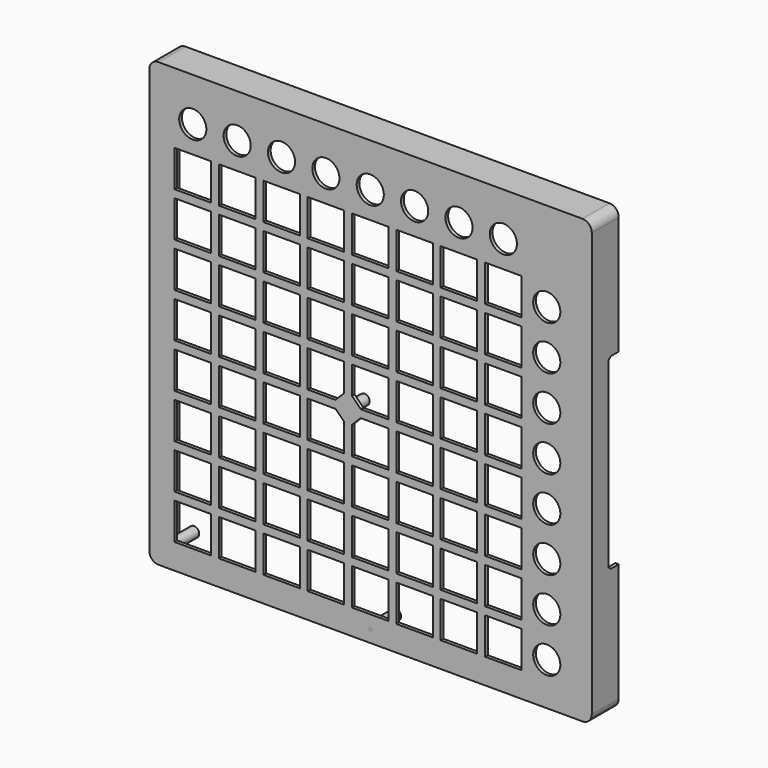
from build123d import *

# Parameters (mm, degrees)
F1_DEPTH  = 18
F0_R      = 2.75
F0_W      = 19.5
F0_H      = 19.5
F0_R_2    = 7.25
F2_DEPTH  = 1.8
F0_R_3    = 0.9
F3_DEPTH  = 17
F4_DEPTH  = 1.8
F0_R_4    = 0.875
F5_DEPTH  = 1.8
F6_DEPTH  = 17
F7_DEPTH  = 1.8
F8_DEPTH  = 17
F9_DEPTH  = 1.8
F10_DEPTH = 17
F12_DEPTH = 325
F13_DEPTH = 17
F14_DEPTH = 1.8
F15_DEPTH = 17
F16_DEPTH = 1.8
F17_W     = 1.5
F17_H     = 11.8
F18_W     = 1.5
F18_H     = 11.8
F19_DEPTH = 0.5
F20_R     = 0.49999


# Not quite as in the source:
# - a fillet or chamfer is up to 0.001 mm smaller than in the source, because OpenCascade refuses the exact size


with BuildPart() as f1:
    # F0 (on Front) → F1 (new body)
    with BuildSketch(Plane.XZ):
        with BuildLine():
            Line((-113.2, -118.2), (113.2, -118.2))
            ThreePointArc((113.2, -118.2), (116.7355339059, -116.7355339059), (118.2, -113.2))
            Line((118.2, -113.2), (118.2, 113.2))
            ThreePointArc((118.2, 113.2), (116.7355339059, 116.7355339059), (113.2, 118.2))
            Line((113.2, 118.2), (-113.2, 118.2))
            ThreePointArc((-113.2, 118.2), (-116.7355339059, 116.7355339059), (-118.2, 113.2))
            Line((-118.2, 113.2), (-118.2, -113.2))
            ThreePointArc((-118.2, -113.2), (-116.7355339059, -116.7355339059), (-113.2, -118.2))
        make_face()
        with BuildLine():
            ThreePointArc((116.4, -111.4), (114.9355339059, -114.9355339059), (111.4, -116.4))
            Line((111.4, -116.4), (-111.4, -116.4))
            ThreePointArc((-111.4, -116.4), (-114.9355339059, -114.9355339059), (-116.4, -111.4))
            Line((-116.4, -111.4), (-116.4, 111.4))
            ThreePointArc((-116.4, 111.4), (-114.9355339059, 114.9355339059), (-111.4, 116.4))
            Line((-111.4, 116.4), (111.4, 116.4))
            ThreePointArc((111.4, 116.4), (114.9355339059, 114.9355339059), (116.4, 111.4))
            Line((116.4, 111.4), (116.4, -111.4))
        make_face(mode=Mode.SUBTRACT)
    extrude(amount=-F1_DEPTH)

    # F0 (on Front) → F2 (join)
    with BuildSketch(Plane.XZ):
        with BuildLine():
            Line((-111.4, -116.4), (111.4, -116.4))
            ThreePointArc((111.4, -116.4), (114.9355339059, -114.9355339059), (116.4, -111.4))
            Line((116.4, -111.4), (116.4, 111.4))
            ThreePointArc((116.4, 111.4), (114.9355339059, 114.9355339059), (111.4, 116.4))
            Line((111.4, 116.4), (-111.4, 116.4))
            ThreePointArc((-111.4, 116.4), (-114.9355339059, 114.9355339059), (-116.4, 111.4))
            Line((-116.4, 111.4), (-116.4, -111.4))
            ThreePointArc((-116.4, -111.4), (-114.9355339059, -114.9355339059), (-111.4, -116.4))
        make_face()
        with Locations((-107.85, -107.85)):
            Circle(F0_R, mode=Mode.SUBTRACT)
        with Locations((-94.95, -94.95)):
            Rectangle(F0_W, F0_H, mode=Mode.SUBTRACT)
        with Locations((-71.25, -94.95)):
            Rectangle(F0_W, F0_H, mode=Mode.SUBTRACT)
        with Locations((-94.95, -71.25)):
            Rectangle(F0_W, F0_H, mode=Mode.SUBTRACT)
        with Locations((-71.25, -71.25)):
            Rectangle(F0_W, F0_H, mode=Mode.SUBTRACT)
        with Locations((-47.55, -94.95)):
            Rectangle(F0_W, F0_H, mode=Mode.SUBTRACT)
        with Locations((-23.85, -94.95)):
            Rectangle(F0_W, F0_H, mode=Mode.SUBTRACT)
        with Locations((-0.1497857198, -94.95)):
            Rectangle(F0_W, F0_H, mode=Mode.SUBTRACT)
        with Locations((-47.55, -71.25)):
            Rectangle(F0_W, F0_H, mode=Mode.SUBTRACT)
        with Locations((-23.85, -71.25)):
            Rectangle(F0_W, F0_H, mode=Mode.SUBTRACT)
        with Locations((-0.1497857198, -71.25)):
            Rectangle(F0_W, F0_H, mode=Mode.SUBTRACT)
        with Locations((-94.95, -47.55)):
            Rectangle(F0_W, F0_H, mode=Mode.SUBTRACT)
        with Locations((-71.25, -47.55)):
            Rectangle(F0_W, F0_H, mode=Mode.SUBTRACT)
        with Locations((-94.95, -23.85)):
            Rectangle(F0_W, F0_H, mode=Mode.SUBTRACT)
        with Locations((-94.95, -0.15)):
            Rectangle(F0_W, F0_H, mode=Mode.SUBTRACT)
        with Locations((-71.25, -23.85)):
            Rectangle(F0_W, F0_H, mode=Mode.SUBTRACT)
        with Locations((-71.25, -0.15)):
            Rectangle(F0_W, F0_H, mode=Mode.SUBTRACT)
        with Locations((-47.55, -47.55)):
            Rectangle(F0_W, F0_H, mode=Mode.SUBTRACT)
        with Locations((-23.85, -47.55)):
            Rectangle(F0_W, F0_H, mode=Mode.SUBTRACT)
        with Locations((-0.1497857198, -47.55)):
            Rectangle(F0_W, F0_H, mode=Mode.SUBTRACT)
        with Locations((-47.55, -23.85)):
            Rectangle(F0_W, F0_H, mode=Mode.SUBTRACT)
        with Locations((-47.55, -0.15)):
            Rectangle(F0_W, F0_H, mode=Mode.SUBTRACT)
        Polygon((9.6002142802, 9.6), (9.6002142802, -9.9), (-5.1834957055, -9.9), (-3.1223304703, -11.9611652352), (-5.2611652352, -14.1), (9.6002142802, -14.1), (9.6002142802, -33.6), (-9.8997857198, -33.6), (-9.8997857198, -18.7386204846), (-11.9611652352, -20.8), (-14.1, -18.6611652352), (-14.1, -33.6), (-33.6, -33.6), (-33.6, -14.1), (-18.6611652352, -14.1), (-20.8, -11.9611652352), (-18.7388347648, -9.9), (-33.6, -9.9), (-33.6, 9.6), (-14.1, 9.6), (-14.1, -5.2611652352), (-11.9611652352, -3.1223304703), (-9.8997857198, -5.1837099858), (-9.8997857198, 9.6), align=None, mode=Mode.SUBTRACT)
        with Locations((0, -111.65)):
            Circle(F0_R, mode=Mode.SUBTRACT)
        with Locations((23.55, -94.95)):
            Rectangle(F0_W, F0_H, mode=Mode.SUBTRACT)
        with Locations((47.25, -94.95)):
            Rectangle(F0_W, F0_H, mode=Mode.SUBTRACT)
        with Locations((23.55, -71.25)):
            Rectangle(F0_W, F0_H, mode=Mode.SUBTRACT)
        with Locations((47.25, -71.25)):
            Rectangle(F0_W, F0_H, mode=Mode.SUBTRACT)
        with Locations((70.95, -94.95)):
            Rectangle(F0_W, F0_H, mode=Mode.SUBTRACT)
        with Locations((107.85, -107.85)):
            Circle(F0_R, mode=Mode.SUBTRACT)
        with Locations((94.15, -95.45)):
            Circle(F0_R_2, mode=Mode.SUBTRACT)
        with Locations((70.95, -71.25)):
            Rectangle(F0_W, F0_H, mode=Mode.SUBTRACT)
        with Locations((94.1499999885, -71.75)):
            Circle(F0_R_2, mode=Mode.SUBTRACT)
        with Locations((23.55, -47.55)):
            Rectangle(F0_W, F0_H, mode=Mode.SUBTRACT)
        with Locations((47.25, -47.55)):
            Rectangle(F0_W, F0_H, mode=Mode.SUBTRACT)
        with Locations((23.55, -23.85)):
            Rectangle(F0_W, F0_H, mode=Mode.SUBTRACT)
        with Locations((23.55, -0.15)):
            Rectangle(F0_W, F0_H, mode=Mode.SUBTRACT)
        with Locations((47.25, -23.85)):
            Rectangle(F0_W, F0_H, mode=Mode.SUBTRACT)
        with Locations((47.25, -0.15)):
            Rectangle(F0_W, F0_H, mode=Mode.SUBTRACT)
        with Locations((70.95, -47.55)):
            Rectangle(F0_W, F0_H, mode=Mode.SUBTRACT)
        with Locations((94.1499999893, -48.05)):
            Circle(F0_R_2, mode=Mode.SUBTRACT)
        with Locations((70.95, -23.85)):
            Rectangle(F0_W, F0_H, mode=Mode.SUBTRACT)
        with Locations((70.95, -0.15)):
            Rectangle(F0_W, F0_H, mode=Mode.SUBTRACT)
        with Locations((94.15, -24.35)):
            Circle(F0_R_2, mode=Mode.SUBTRACT)
        with Locations((94.15, -0.65)):
            Circle(F0_R_2, mode=Mode.SUBTRACT)
        with Locations((-94.95, 23.55)):
            Rectangle(F0_W, F0_H, mode=Mode.SUBTRACT)
        with Locations((-71.25, 23.55)):
            Rectangle(F0_W, F0_H, mode=Mode.SUBTRACT)
        with Locations((-94.95, 47.25)):
            Rectangle(F0_W, F0_H, mode=Mode.SUBTRACT)
        with Locations((-71.25, 47.25)):
            Rectangle(F0_W, F0_H, mode=Mode.SUBTRACT)
        with Locations((-47.55, 23.55)):
            Rectangle(F0_W, F0_H, mode=Mode.SUBTRACT)
        with Locations((-23.85, 23.55)):
            Rectangle(F0_W, F0_H, mode=Mode.SUBTRACT)
        with Locations((-0.1497857198, 23.55)):
            Rectangle(F0_W, F0_H, mode=Mode.SUBTRACT)
        with Locations((-47.55, 47.25)):
            Rectangle(F0_W, F0_H, mode=Mode.SUBTRACT)
        with Locations((-23.85, 47.25)):
            Rectangle(F0_W, F0_H, mode=Mode.SUBTRACT)
        with Locations((-0.15, 47.25)):
            Rectangle(F0_W, F0_H, mode=Mode.SUBTRACT)
        with Locations((-94.95, 70.95)):
            Rectangle(F0_W, F0_H, mode=Mode.SUBTRACT)
        with Locations((-71.25, 70.95)):
            Rectangle(F0_W, F0_H, mode=Mode.SUBTRACT)
        with Locations((-94.95, 94.95)):
            Circle(F0_R_2, mode=Mode.SUBTRACT)
        with Locations((-107.85, 107.85)):
            Circle(F0_R, mode=Mode.SUBTRACT)
        with Locations((-71.25, 94.95)):
            Circle(F0_R_2, mode=Mode.SUBTRACT)
        with Locations((-47.55, 70.95)):
            Rectangle(F0_W, F0_H, mode=Mode.SUBTRACT)
        with Locations((-23.85, 70.95)):
            Rectangle(F0_W, F0_H, mode=Mode.SUBTRACT)
        with Locations((-0.15, 70.95)):
            Rectangle(F0_W, F0_H, mode=Mode.SUBTRACT)
        with Locations((-47.55, 94.9499985917)):
            Circle(F0_R_2, mode=Mode.SUBTRACT)
        with Locations((-23.85, 94.9499985917)):
            Circle(F0_R_2, mode=Mode.SUBTRACT)
        with Locations((-0.15, 94.95)):
            Circle(F0_R_2, mode=Mode.SUBTRACT)
        with Locations((23.55, 23.55)):
            Rectangle(F0_W, F0_H, mode=Mode.SUBTRACT)
        with Locations((47.25, 23.55)):
            Rectangle(F0_W, F0_H, mode=Mode.SUBTRACT)
        with Locations((23.55, 47.25)):
            Rectangle(F0_W, F0_H, mode=Mode.SUBTRACT)
        with Locations((47.25, 47.25)):
            Rectangle(F0_W, F0_H, mode=Mode.SUBTRACT)
        with Locations((70.95, 23.55)):
            Rectangle(F0_W, F0_H, mode=Mode.SUBTRACT)
        with Locations((94.1499999896, 23.05)):
            Circle(F0_R_2, mode=Mode.SUBTRACT)
        with Locations((70.95, 47.25)):
            Rectangle(F0_W, F0_H, mode=Mode.SUBTRACT)
        with Locations((94.15, 46.75)):
            Circle(F0_R_2, mode=Mode.SUBTRACT)
        with Locations((23.55, 70.95)):
            Rectangle(F0_W, F0_H, mode=Mode.SUBTRACT)
        with Locations((47.25, 70.95)):
            Rectangle(F0_W, F0_H, mode=Mode.SUBTRACT)
        with Locations((23.55, 94.95)):
            Circle(F0_R_2, mode=Mode.SUBTRACT)
        with Locations((0, 111.65)):
            Circle(F0_R, mode=Mode.SUBTRACT)
        with Locations((47.25, 94.95)):
            Circle(F0_R_2, mode=Mode.SUBTRACT)
        with Locations((70.95, 70.95)):
            Rectangle(F0_W, F0_H, mode=Mode.SUBTRACT)
        with Locations((94.15, 70.45)):
            Circle(F0_R_2, mode=Mode.SUBTRACT)
        with Locations((70.95, 94.95)):
            Circle(F0_R_2, mode=Mode.SUBTRACT)
        with Locations((107.85, 107.85)):
            Circle(F0_R, mode=Mode.SUBTRACT)
        Polygon((-14.1, -9.9), (-14.1, -5.2611652352), (-18.7388347648, -9.9), align=None)
        Polygon((-3.1223304703, -11.9611652352), (-5.1834957055, -9.9), (-9.8997857198, -9.9), (-9.8997857198, -5.1837099858), (-11.9611652352, -3.1223304703), (-14.1, -5.2611652352), (-14.1, -9.9), (-18.7388347648, -9.9), (-20.8, -11.9611652352), (-18.6611652352, -14.1), (-14.1, -14.1), (-14.1, -18.6611652352), (-11.9611652352, -20.8), (-9.8997857198, -18.7386204846), (-9.8997857198, -14.1), (-5.2611652352, -14.1), align=None)
        with Locations((-12, -12)):
            Circle(F0_R, mode=Mode.SUBTRACT)
        Polygon((-18.6611652352, -14.1), (-14.1, -18.6611652352), (-14.1, -14.1), align=None)
        Polygon((-9.8997857198, -18.7386204846), (-5.2611652352, -14.1), (-9.8997857198, -14.1), align=None)
        Polygon((-9.8997857198, -9.9), (-5.1834957055, -9.9), (-9.8997857198, -5.1837099858), align=None)
    extrude(amount=-F2_DEPTH)

    # F0 (on Front) → F3 (join)
    with BuildSketch(Plane.XZ):
        with Locations((-12, -12)):
            Circle(F0_R)
        with Locations((-12, -12)):
            Circle(F0_R_3, mode=Mode.SUBTRACT)
    extrude(amount=-F3_DEPTH)

    # F0 (on Front) → F4 (join)
    with BuildSketch(Plane.XZ):
        with Locations((-12, -12)):
            Circle(F0_R_3)
    extrude(amount=-F4_DEPTH)

    # F0 (on Front) → F6 (join)
    with BuildSketch(Plane.XZ):
        with Locations((0, 111.65)):
            Circle(F0_R)
        with Locations((0, 111.65)):
            Circle(F0_R_4, mode=Mode.SUBTRACT)
    extrude(amount=-F6_DEPTH)

    # F0 (on Front) → F7 (join)
    with BuildSketch(Plane.XZ):
        with Locations((0, 111.65)):
            Circle(F0_R_4)
    extrude(amount=-F7_DEPTH)

    # F0 (on Front) → F8 (join)
    with BuildSketch(Plane.XZ):
        with Locations((107.85, -107.85)):
            Circle(F0_R)
        with Locations((107.85, -107.85)):
            Circle(F0_R_4, mode=Mode.SUBTRACT)
    extrude(amount=-F8_DEPTH)

    # F0 (on Front) → F9 (join)
    with BuildSketch(Plane.XZ):
        with Locations((107.85, -107.85)):
            Circle(F0_R_4)
    extrude(amount=-F9_DEPTH)

    # F0 (on Front) → F10 (join)
    with BuildSketch(Plane.XZ):
        with Locations((0, -111.65)):
            Circle(F0_R)
        with Locations((0, -111.65)):
            Circle(F0_R_4, mode=Mode.SUBTRACT)
    extrude(amount=-F10_DEPTH)

    # F11 (on face) → F12 (cut)
    with BuildSketch(Plane.YZ.offset(118.2)):
        with BuildLine():
            Line((18, -50), (18, 50))
            Line((18, 50), (13.5, 50))
            ThreePointArc((13.5, 50), (11.732233047, 49.267766953), (11, 47.5))
            Line((11, 47.5), (11, -47.5))
            ThreePointArc((11, -47.5), (11.732233047, -49.267766953), (13.5, -50))
            Line((13.5, -50), (18, -50))
        make_face()
    extrude(amount=-F12_DEPTH, mode=Mode.SUBTRACT)

    # F0 (on Front) → F13 (join)
    with BuildSketch(Plane.XZ):
        with Locations((107.85, 107.85)):
            Circle(F0_R)
        with Locations((107.85, 107.85)):
            Circle(F0_R_4, mode=Mode.SUBTRACT)
    extrude(amount=-F13_DEPTH)

    # F0 (on Front) → F14 (join)
    with BuildSketch(Plane.XZ):
        with Locations((107.85, 107.85)):
            Circle(F0_R_4)
    extrude(amount=-F14_DEPTH)

    # F0 (on Front) → F15 (join)
    with BuildSketch(Plane.XZ):
        with Locations((-107.85, -107.85)):
            Circle(F0_R)
        with Locations((-107.85, -107.85)):
            Circle(F0_R_4, mode=Mode.SUBTRACT)
        with Locations((-107.85, 107.85)):
            Circle(F0_R)
        with Locations((-107.85, 107.85)):
            Circle(F0_R_4, mode=Mode.SUBTRACT)
    extrude(amount=-F15_DEPTH)

    # F0 (on Front) → F16 (join)
    with BuildSketch(Plane.XZ):
        with Locations((-107.85, -107.85)):
            Circle(F0_R_4)
        with Locations((-107.85, 107.85)):
            Circle(F0_R_4)
    extrude(amount=-F16_DEPTH)

    # F17 (on face) + F18 (on face) → F19 (join, symmetric)
    with BuildSketch(Plane(origin=(116.4, 0, 0), x_dir=(0, -1, 0), z_dir=(-1, 0, 0))):
        with Locations((-7.95, 26.3)):
            Rectangle(F17_W, F17_H)
        with Locations((-7.95, -26.3)):
            Rectangle(F17_W, F17_H)
    with BuildSketch(Plane.YZ.offset(-116.4)):
        with Locations((8.8734421776, 26.3)):
            Rectangle(F18_W, F18_H)
        with Locations((8.8734421776, -26.3)):
            Rectangle(F18_W, F18_H)
    extrude(amount=F19_DEPTH, both=True, dir=(-1, 0, 0))

    # F20 (radius 0.5 in the source; OpenCascade refuses exactly that, so slightly less here)
    f20_edges = [f1.edges().sort_by_distance(p)[0] for p in [
        (115.9, 7.95, 32.2),
        (115.9, 8.7, 26.3),
        (115.9, 7.95, 20.4),
        (115.9, 7.2, 26.3),
        (115.9, 7.95, -20.4),
        (115.9, 8.7, -26.3),
        (115.9, 7.95, -32.2),
        (115.9, 7.2, -26.3),
        (116.15, 8.7, -32.2),
        (116.15, 7.2, -32.2),
        (116.15, 7.2, -20.4),
        (116.15, 8.7, -20.4),
        (116.15, 8.7, 32.2),
        (116.15, 7.2, 32.2),
        (116.15, 8.7, 20.4),
        (116.15, 7.2, 20.4),
        (-115.9, 8.873442, 32.2),
        (-115.9, 8.123442, 26.3),
        (-115.9, 8.873442, 20.4),
        (-115.9, 9.623442, 26.3),
        (-115.9, 8.873442, -20.4),
        (-115.9, 8.123442, -26.3),
        (-115.9, 8.873442, -32.2),
        (-115.9, 9.623442, -26.3),
        (-116.15, 9.623442, -20.4),
        (-116.15, 9.623442, -32.2),
        (-116.15, 8.123442, -32.2),
        (-116.15, 8.123442, -20.4),
        (-116.15, 8.123442, 20.4),
        (-116.15, 9.623442, 20.4),
        (-116.15, 9.623442, 32.2),
        (-116.15, 8.123442, 32.2),
    ]]
    fillet(f20_edges, radius=F20_R)


with BuildPart() as f5:
    # F0 (on Front) → F5 (new body)
    with BuildSketch(Plane.XZ):
        with Locations((0, -111.65)):
            Circle(F0_R_4)
    extrude(amount=-F5_DEPTH)


solid = Compound([f1.part, f5.part])
